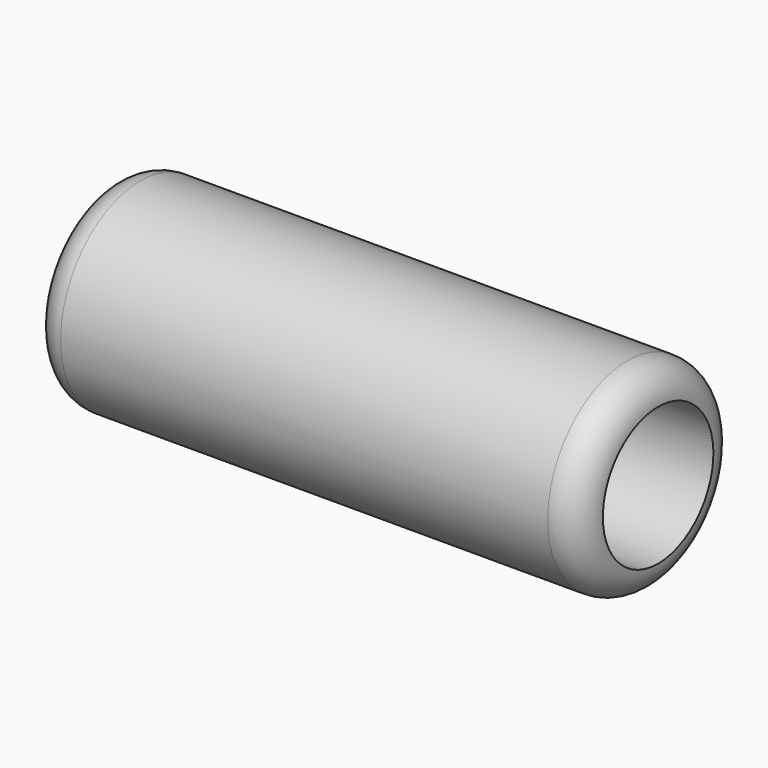
from build123d import *

# Parameters (mm, degrees)
F3_R = 6.35


# Not quite as in the source:
# - a fillet or chamfer that OpenCascade refuses, or shapes differently, is made with other operations: its cross-section is extruded or revolved along the edge and cut away or added


with BuildPart() as f1:
    # F0 (on Front) → F1 (revolve)
    with BuildSketch(Plane.XZ):
        Polygon((-75.2320736647, 15.875), (-75.2320736647, 0), (38.2805263353, 0), (38.2805263353, 6.35), (-71.0156736647, 6.35), (-71.2696736647, 6.35), (-71.2696736647, 15.875), align=None)
    revolve(axis=Axis((-17.1681363136, 0, 20.6502), (1, 0, 0)))

    # F2: fillet of radius 6.35 on 2 edges, made by hand

    # F2_s1 → F2_t2 (revolve, cut)
    with BuildSketch(Plane.XZ):
        with BuildLine():
            ThreePointArc((31.9305263353, 0), (36.4206543959, 1.8598719395), (38.2805263353, 6.35))
            Line((38.2805263353, 6.35), (38.2805263353, 0))
            Line((38.2805263353, 0), (31.9305263353, 0))
        make_face()
    revolve(axis=Axis((38.2805263353, 0, 20.6502), (1, 0, 0)), mode=Mode.SUBTRACT)

    # F2_s3 → F2_t4 (revolve, cut)
    with BuildSketch(Plane.XZ):
        with BuildLine():
            ThreePointArc((-71.2696736647, 9.9909651395), (-72.3526175609, 13.5378821106), (-75.2320736647, 15.875))
            Line((-75.2320736647, 15.875), (-71.2696736647, 15.875))
            Line((-71.2696736647, 15.875), (-71.2696736647, 9.9909651395))
        make_face()
    revolve(axis=Axis((-71.2696736647, 0, 20.6502), (1, 0, 0)), mode=Mode.SUBTRACT)

    # F3
    f3_edges = [f1.edges().sort_by_distance(p)[0] for p in [
        (-75.232074, 0, 41.3004),
    ]]
    fillet(f3_edges, radius=F3_R)


solid = f1.part
